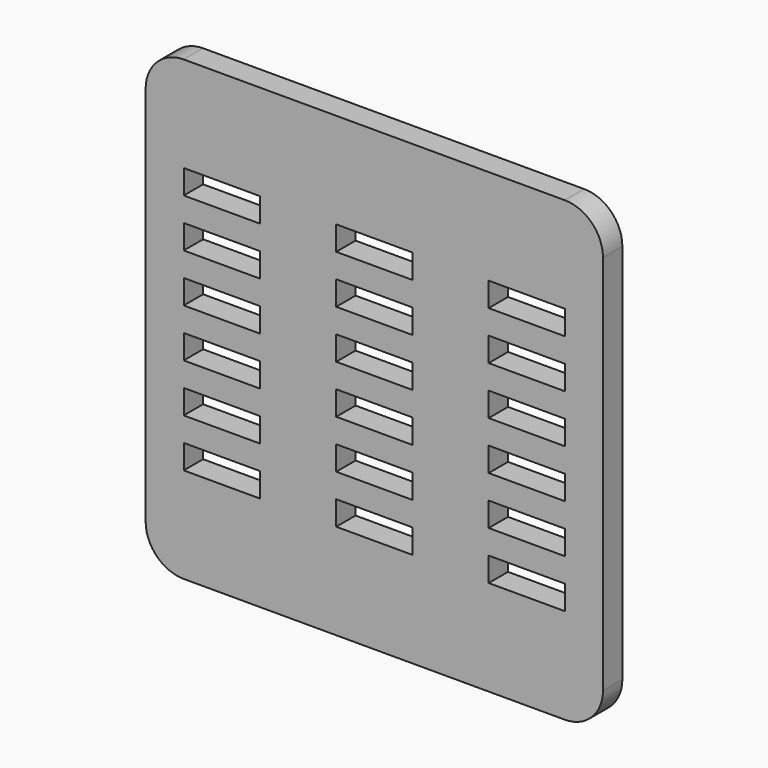
from build123d import *

# Parameters (mm, degrees)
F0_W     = 60
F0_H     = 60
F1_DEPTH = 3.175
F2_W     = 10
F2_H     = 3.175
F3_DEPTH = 3.176
F4_R     = 5


# Not quite as in the source:
# - a length typed as a fraction of an inch, garbled in the dataset ("3 / 203.2 mm" for 3/8 in), is restored


with BuildPart() as f1:
    # F0 (on Front) → F1 (new body)
    with BuildSketch(Plane.XZ):
        Rectangle(F0_W, F0_H)
    extrude(amount=F1_DEPTH)

    # F2 (on face) → F3 (cut, through all)
    with BuildSketch(Plane.XZ.offset(3.175)):
        with Locations((-20, -15.875)):
            Rectangle(F2_W, F2_H)
        with Locations((0, -15.875)):
            Rectangle(F2_W, F2_H)
        with Locations((20, -15.875)):
            Rectangle(F2_W, F2_H)
        with Locations((-20, -9.525)):
            Rectangle(F2_W, F2_H)
        with Locations((0, -9.525)):
            Rectangle(F2_W, F2_H)
        with Locations((20, -9.525)):
            Rectangle(F2_W, F2_H)
        with Locations((-20, -3.175)):
            Rectangle(F2_W, F2_H)
        with Locations((0, -3.175)):
            Rectangle(F2_W, F2_H)
        with Locations((20, -3.175)):
            Rectangle(F2_W, F2_H)
        with Locations((-20, 3.175)):
            Rectangle(F2_W, F2_H)
        with Locations((0, 3.175)):
            Rectangle(F2_W, F2_H)
        with Locations((20, 3.175)):
            Rectangle(F2_W, F2_H)
        with Locations((-20, 9.525)):
            Rectangle(F2_W, F2_H)
        with Locations((0, 9.525)):
            Rectangle(F2_W, F2_H)
        with Locations((20, 9.525)):
            Rectangle(F2_W, F2_H)
        with Locations((-20, 15.875)):
            Rectangle(F2_W, F2_H)
        with Locations((0, 15.875)):
            Rectangle(F2_W, F2_H)
        with Locations((20, 15.875)):
            Rectangle(F2_W, F2_H)
    extrude(amount=-F3_DEPTH, mode=Mode.SUBTRACT)

    # F4
    f4_edges = [f1.edges().sort_by_distance(p)[0] for p in [
        (-30, -1.5875, 30),
        (30, -1.5875, 30),
        (-30, -1.5875, -30),
        (30, -1.5875, -30),
    ]]
    fillet(f4_edges, radius=F4_R)


solid = f1.part
